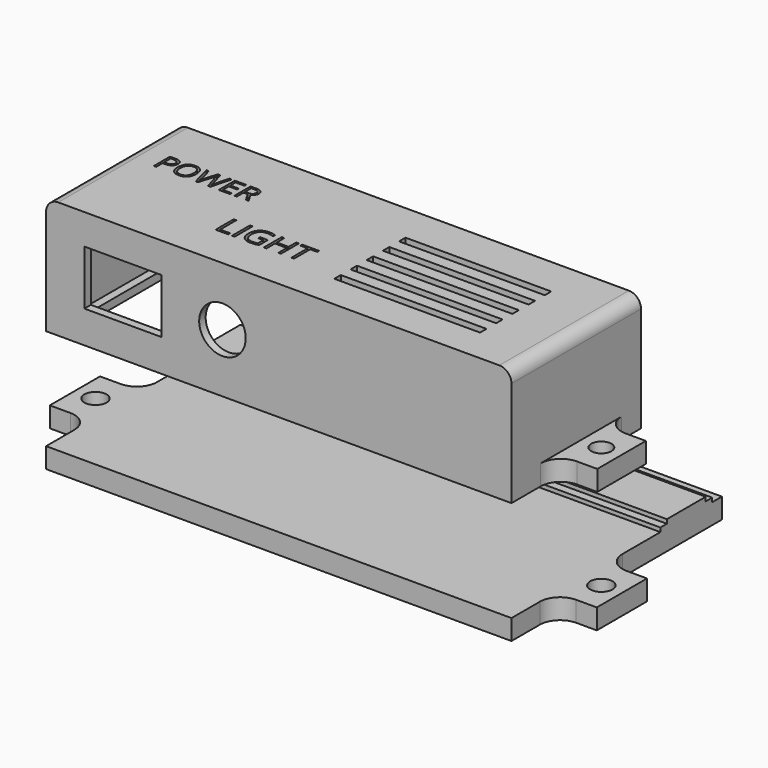
from build123d import *

# Parameters (mm, degrees)
F0_W            = 111
F0_H            = 36
F1_DEPTH        = 25
F2_DEPTH        = 3
F3_W            = 115
F3_H            = 40
F4_DEPTH        = 2
F6_DEPTH        = 2
F7_R            = 2.5
F8_DEPTH        = 10
F9_R            = 2.5
F10_DEPTH       = 10
F12_DEPTH       = 5
F13_R           = 5.75
F14_DEPTH       = 5
F15_R           = 5
F16_R           = 3
F17_W           = 36
F17_H           = 2
F18_DEPTH       = 5
F19_W           = 107
F19_H           = 32
F20_DEPTH       = 5
F21_TEXT_SIZE   = 6.9575869323
F21_TEXT_SIZE_2 = 7.7998362637
F22_DEPTH       = 5
F25_DEPTH       = 5
F26_R           = 5
F27_R           = 2.75
F28_DEPTH       = 6
F29_W           = 115
F29_H           = 2
F30_DEPTH       = 1
F29_H_2         = 12
F31_DEPTH       = 2
F32_R           = 2.75
F33_DEPTH       = 10


# Not quite as in the source:
# - Text() gives the source's letters only with a copy of the font that has no kerning and outlines rounded to 1/6400 em; it was checked with that copy


with BuildPart() as f1:
    # F0 (on Top) → F1 (new body)
    with BuildSketch(Plane.XY):
        Polygon((0, 14), (0, 0), (115, 0), (115, 14), (115, 29), (115, 40), (0, 40), (0, 29), align=None)
        with Locations((57.5, 20)):
            Rectangle(F0_W, F0_H, mode=Mode.SUBTRACT)
    extrude(amount=F1_DEPTH)

    # F0 (on Top) → F2 (join)
    with BuildSketch(Plane.XY):
        Polygon((-10, 14), (0, 14), (0, 29), (-10, 29), (-10, 20), align=None)
        Polygon((115, 29), (115, 14), (125, 14), (125, 15), (125, 29), align=None)
    extrude(amount=F2_DEPTH)

    # F3 (on face) → F4 (join)
    with BuildSketch(Plane.XY.offset(25)):
        with Locations((57.5, 20)):
            Rectangle(F3_W, F3_H)
    extrude(amount=F4_DEPTH)

    # F5 (on face) → F6 (join)
    with BuildSketch(Plane(origin=(0, 0, 0), x_dir=(1, 0, 0), z_dir=(0, 0, -1))):
        Polygon((115, 0), (0, 0), (0, -14), (-10, -14), (-10, -29), (0, -29), (0, -40), (115, -40), (115, -29), (125, -29), (125, -14), (115, -14), align=None)
    extrude(amount=F6_DEPTH)

    # F7 (on face) → F8 (cut)
    with BuildSketch(Plane.XY.offset(3)):
        with Locations((-5, 21.5)):
            Circle(F7_R)
    extrude(amount=-F8_DEPTH, mode=Mode.SUBTRACT)

    # F9 (on face) → F10 (cut)
    with BuildSketch(Plane.XY.offset(3)):
        with Locations((120, 21.5)):
            Circle(F9_R)
    extrude(amount=-F10_DEPTH, mode=Mode.SUBTRACT)

    # F11 (on face) → F12 (cut)
    with BuildSketch(Plane.XZ):
        Polygon((28.4624864608, 19.5), (18.4624864608, 19.5), (9.4624864608, 19.5), (9.4624864608, 6), (28.4624864608, 6), align=None)
    extrude(amount=-F12_DEPTH, mode=Mode.SUBTRACT)

    # F13 (on face) → F14 (cut)
    with BuildSketch(Plane.XZ):
        with Locations((43.5828566551, 12.5)):
            Circle(F13_R)
    extrude(amount=-F14_DEPTH, mode=Mode.SUBTRACT)

    # F15
    f15_edges = [f1.edges().sort_by_distance(p)[0] for p in [
        (0, 14, 0.5),
        (0, 29, 0.5),
        (115, 14, 0.5),
        (115, 29, 0.5),
    ]]
    fillet(f15_edges, radius=F15_R)

    # F16
    f16_edges = [f1.edges().sort_by_distance(p)[0] for p in [
        (0, 20, 27),
        (115, 20, 27),
    ]]
    fillet(f16_edges, radius=F16_R)

    # F17 (on face) → F18 (cut)
    with BuildSketch(Plane.XY.offset(27)):
        with Locations((82.5320262313, 29.3591875583)):
            Rectangle(F17_W, F17_H)
        with Locations((82.5320262313, 24.3591875583)):
            Rectangle(F17_W, F17_H)
        with Locations((82.5320262313, 19.3591875583)):
            Rectangle(F17_W, F17_H)
        with Locations((82.5320262313, 14.3591875583)):
            Rectangle(F17_W, F17_H)
        with Locations((82.5320262313, 9.3591875583)):
            Rectangle(F17_W, F17_H)
    extrude(amount=-F18_DEPTH, mode=Mode.SUBTRACT)

    # F19 (on face) → F20 (cut)
    with BuildSketch(Plane(origin=(0, 0, -2), x_dir=(1, 0, 0), z_dir=(0, 0, -1))):
        with Locations((57.5, -20)):
            Rectangle(F19_W, F19_H)
    extrude(amount=-F20_DEPTH, mode=Mode.SUBTRACT)

    # F21 (on face) → F22 (cut)
    with BuildSketch(Plane.XY.offset(27)):
        with Locations((7.2130723856, 23.4243269078)):
            Text('POWER', F21_TEXT_SIZE, font='Open Sans', text_align=(TextAlign.LEFT, TextAlign.BOTTOM))
        with Locations((33.0800078809, 10.0686750375)):
            Text('LIGHT', F21_TEXT_SIZE_2, font='Open Sans', text_align=(TextAlign.LEFT, TextAlign.BOTTOM))
    extrude(amount=-F22_DEPTH, mode=Mode.SUBTRACT)


with BuildPart() as f25:
    # F24 (on offset) → F25 (new body)
    with BuildSketch(Plane(origin=(0, 0, -27), x_dir=(1, 0, 0), z_dir=(0, 0, -1))):
        Polygon((115, 0), (0, 0), (0, -13.7558626011), (-10.0820660591, -13.7558626011), (-10.0820660591, -29.265826568), (0, -29.265826568), (0, -65), (115, -65), (115, -29.265826568), (125.0762045383, -29.265826568), (125.0762045383, -13.7558626011), (115, -13.7558626011), align=None)
    extrude(amount=F25_DEPTH)

    # F26
    f26_edges = [f25.edges().sort_by_distance(p)[0] for p in [
        (0, 29.265827, -29.5),
        (0, 13.755863, -29.5),
        (115, 29.265827, -29.5),
        (115, 13.755863, -29.5),
    ]]
    fillet(f26_edges, radius=F26_R)

    # F27 (on face) → F28 (cut)
    with BuildSketch(Plane(origin=(0, 0, -32), x_dir=(1, 0, 0), z_dir=(0, 0, -1))):
        with Locations((-5, -21.5108445846)):
            Circle(F27_R)
        with Locations((120, -21.5108445846)):
            Circle(F27_R)
    extrude(amount=-F28_DEPTH, mode=Mode.SUBTRACT)

    # F29 (on face) → F30 (join)
    with BuildSketch(Plane.XY.offset(-27)):
        with Locations((57.5, 61)):
            Rectangle(F29_W, F29_H)
        with Locations((57.5, 47)):
            Rectangle(F29_W, F29_H)
    extrude(amount=F30_DEPTH)

    # F29 (on face) → F31 (join)
    with BuildSketch(Plane.XY.offset(-27)):
        with Locations((57.5, 54)):
            Rectangle(F29_W, F29_H_2)
    extrude(amount=F31_DEPTH)

    # F32 (on face) → F33 (cut)
    with BuildSketch(Plane.XY.offset(-25)):
        with Locations((90, 54)):
            Circle(F32_R)
        with Locations((25, 54)):
            Circle(F32_R)
    extrude(amount=-F33_DEPTH, mode=Mode.SUBTRACT)


solid = Compound([f1.part, f25.part])
